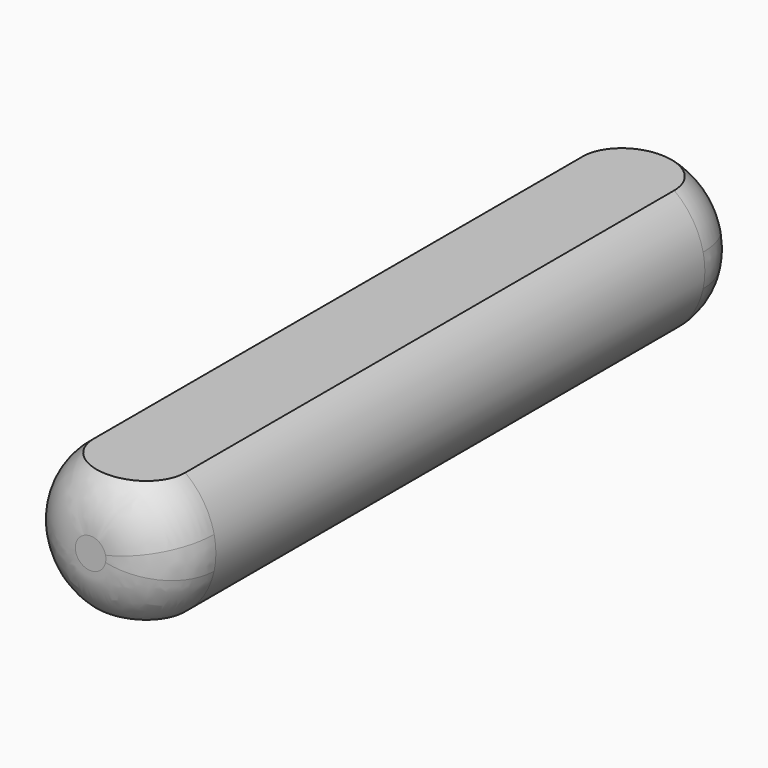
from build123d import *

# Parameters (mm, degrees)
F1_DEPTH    = 24
F2_T2_ANGLE = 335.5716732895
F2_T4_ANGLE = 335.5716732895
F2_T6_ANGLE = 253.6182255886
F2_T8_ANGLE = 253.6182255886


# Not quite as in the source:
# - a fillet or chamfer that OpenCascade refuses, or shapes differently, is made with other operations: its cross-section is extruded or revolved along the edge and cut away or added


with BuildPart() as f1:
    # F0 (on Front) → F1 (new body)
    with BuildSketch(Plane.XZ):
        with BuildLine():
            Line((1.5, 2), (-1.5, 2))
            ThreePointArc((-1.5, 2), (-2.5, 0), (-1.5, -2))
            Line((-1.5, -2), (1.5, -2))
            ThreePointArc((1.5, -2), (2.5, 0), (1.5, 2))
        make_face()
    extrude(amount=F1_DEPTH)

    # F2: fillet of radius 2 on 4 edges, made by hand

    # F2_s1 → F2_t2 (revolve, cut)
    with BuildSketch(Plane(origin=(0, 0, 0), x_dir=(0, 1, 0), z_dir=(0.2115664045, 0, -0.9773636255))):
        with BuildLine():
            ThreePointArc((-2, 2.5), (-0.5857864376, 1.9142135624), (0, 0.5))
            Line((0, 0.5), (0, 2.5))
            Line((0, 2.5), (-2, 2.5))
        make_face()
    revolve(axis=Axis((0, 0, 0), (0, -1, 0)), revolution_arc=F2_T2_ANGLE, mode=Mode.SUBTRACT)

    # F2_s3 → F2_t4 (revolve, cut)
    with BuildSketch(Plane(origin=(0, 0, 0), x_dir=(0, 1, 0), z_dir=(0.2115664045, 0, -0.9773636255))):
        with BuildLine():
            ThreePointArc((-22, 2.5), (-23.4142135624, 1.9142135624), (-24, 0.5))
            Line((-24, 0.5), (-24, 2.5))
            Line((-24, 2.5), (-22, 2.5))
        make_face()
    revolve(axis=Axis((0, -24, 0), (0, -1, 0)), revolution_arc=F2_T4_ANGLE, mode=Mode.SUBTRACT)

    # F2_s5 → F2_t6 (revolve, cut)
    with BuildSketch(Plane(origin=(0, 0, 0), x_dir=(0, 1, 0), z_dir=(-0.8006360872, 0, 0.5991509459))):
        with BuildLine():
            ThreePointArc((-2, 2.5), (-0.5857864376, 1.9142135624), (0, 0.5))
            Line((0, 0.5), (0, 2.5))
            Line((0, 2.5), (-2, 2.5))
        make_face()
    revolve(axis=Axis((0, 0, 0), (0, -1, 0)), revolution_arc=F2_T6_ANGLE, mode=Mode.SUBTRACT)

    # F2_s7 → F2_t8 (revolve, cut)
    with BuildSketch(Plane(origin=(0, 0, 0), x_dir=(0, 1, 0), z_dir=(-0.8006360872, 0, 0.5991509459))):
        with BuildLine():
            ThreePointArc((-22, 2.5), (-23.4142135624, 1.9142135624), (-24, 0.5))
            Line((-24, 0.5), (-24, 2.5))
            Line((-24, 2.5), (-22, 2.5))
        make_face()
    revolve(axis=Axis((0, -24, 0), (0, -1, 0)), revolution_arc=F2_T8_ANGLE, mode=Mode.SUBTRACT)


solid = f1.part
